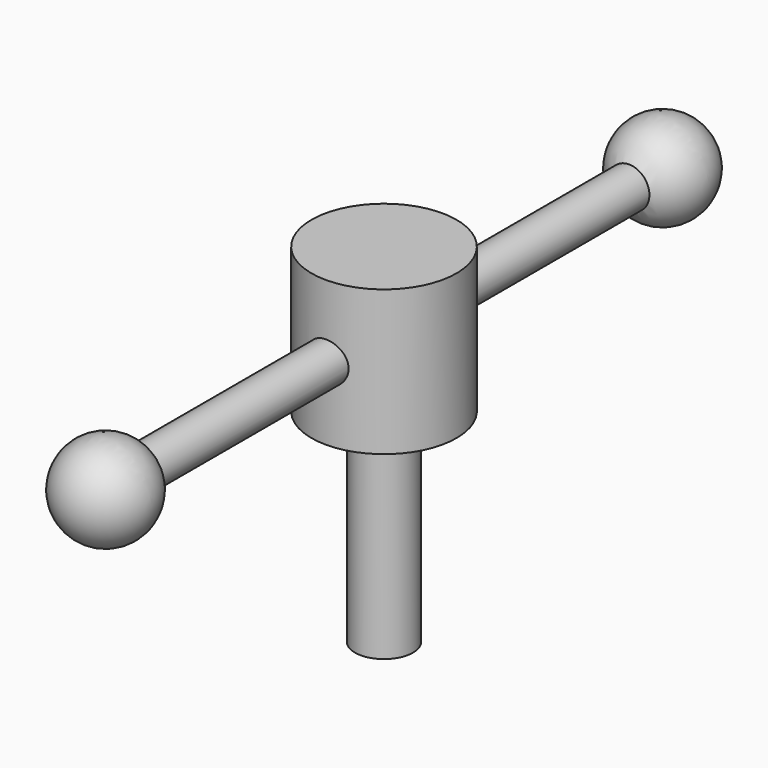
from build123d import *

# Parameters (mm, degrees)
F2_R     = 4.445
F3_DEPTH = 76.2


with BuildPart() as f1:
    # F0 (on Right) → F1 (revolve)
    with BuildSketch(Plane.YZ):
        Polygon((-6.35, 0), (0, 0), (0, 76.2), (-15.875, 76.2), (-15.875, 44.45), (-6.35, 44.45), align=None)
    revolve(axis=Axis((0, 0, 38.1), (0, 0, 1)))

    # F2 (on Front) → F3 (join, symmetric)
    with BuildSketch(Plane.XZ):
        with Locations((0, 60.325)):
            Circle(F2_R)
    extrude(amount=F3_DEPTH, both=True)

    # F4 (on face) → F5 (revolve)
    with BuildSketch(Plane(origin=(0, 76.2, 0), x_dir=(-1, 0, 0), z_dir=(0, 1, 0))):
        with BuildLine():
            ThreePointArc((10.16, 60.325), (0, 70.485), (-10.16, 60.325))
            Line((-10.16, 60.325), (-4.445, 60.325))
            ThreePointArc((-4.445, 60.325), (0, 64.77), (4.445, 60.325))
            Line((4.445, 60.325), (10.16, 60.325))
        make_face()
        with BuildLine():
            ThreePointArc((4.445, 60.325), (0, 64.77), (-4.445, 60.325))
            Line((-4.445, 60.325), (4.445, 60.325))
        make_face()
    revolve(axis=Axis((0, 76.2, 60.325), (-1, 0, 0)))

    # F6 (on face) → F7 (revolve)
    with BuildSketch(Plane.XZ.offset(76.2)):
        with BuildLine():
            ThreePointArc((10.16, 60.325), (0, 70.485), (-10.16, 60.325))
            Line((-10.16, 60.325), (10.16, 60.325))
        make_face()
    revolve(axis=Axis((0, -76.2, 60.325), (1, 0, 0)))


solid = f1.part
